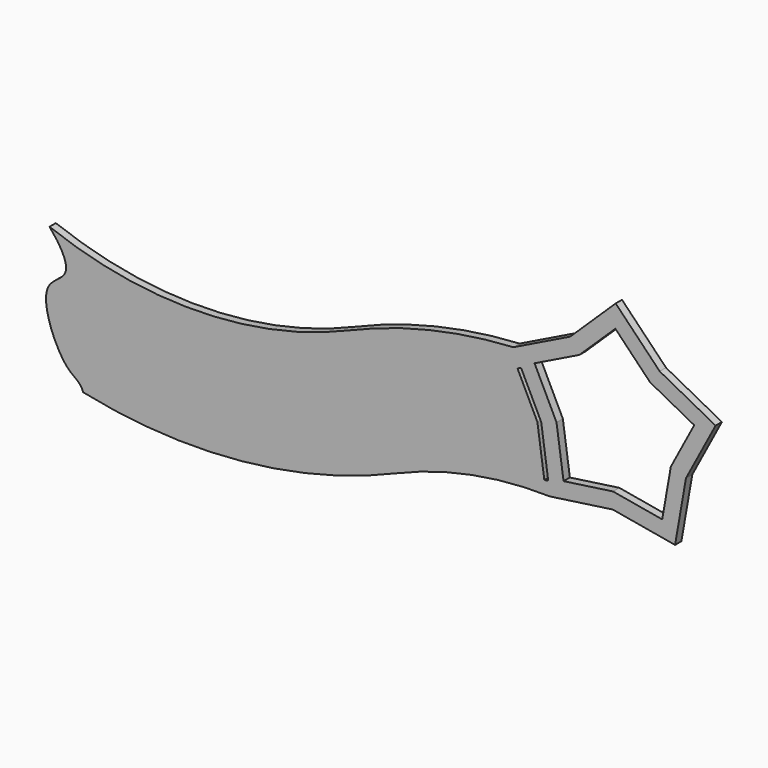
from build123d import *

# Parameters (mm, degrees)
F1_DEPTH = 3.175
F3_DEPTH = 25.4


# Not quite as in the source:
# - a feature of the source that left no trace in its solid (it failed there, or was rolled back) is left out


with BuildPart() as f1:
    # F0 (on Front) → F1 (new body)
    with BuildSketch(Plane.XZ):
        Polygon((83.7385465681, 60.7950414864), (65.4867140893, 43.1201200129), (42.6659945136, 31.9511005402), (48.4525043638, 20.1278488249), (53.8348904797, 9.1303205178), (53.9749918148, 8.1434892953), (55.6890408221, -3.9297509459), (57.4061805077, -16.0247609861), (82.5613006616, -12.4537432078), (107.5886724448, -16.8312881314), (111.9661336404, 8.1960982966), (123.863112913, 30.645911706), (101.4134680417, 42.5432090075), align=None)
        Polygon((62.8005820601, -8.8453070311), (59.98049806, 11.018507533), (51.1609480861, 29.0390003787), (69.1816050409, 37.8587515602), (83.5943604063, 51.8159429598), (97.5514190703, 37.4033246624), (115.278932926, 28.0085434102), (105.884368679, 10.2808320666), (102.427683451, -9.4821750964), (82.6646160624, -6.0254111952), align=None, mode=Mode.SUBTRACT)
        with BuildLine():
            Line((48.4525043638, 20.1278488249), (42.6659945136, 31.9511005402))
            ThreePointArc((42.6659945136, 31.9511005402), (8.9754555579, 27.0708614751), (-23.3620781244, 16.433518583))
            ThreePointArc((-23.3620781244, 16.433518583), (-83.2539454778, 3.5037557836), (-143.6249151078, 13.9708741582))
            add(Edge.make_bspline(
                [(-143.6249151078, 13.9708741582), (-139.3821490751, 9.1987873198), (-135.7140854359, 2.9639524936), (-137.4607610868, -0.5827256571), (-137.6279600012, -0.8521879559)],
                knots=[0, 0, 0, 0, 0.2240060147, 0.243416319, 0.243416319, 0.243416319, 0.243416319], degree=3))
            ThreePointArc((-137.6279600012, -0.8521879559), (-77.5676001001, -8.3586658465), (-18.6118863058, 5.3459995187))
            ThreePointArc((-18.6118863058, 5.3459995187), (14.224158407, 15.8953190594), (48.4525043638, 20.1278488249))
        make_face()
        with BuildLine():
            Line((53.8348904797, 9.1303205178), (48.4525043638, 20.1278488249))
            ThreePointArc((48.4525043638, 20.1278488249), (14.224158407, 15.8953190594), (-18.6118863058, 5.3459995187))
            ThreePointArc((-18.6118863058, 5.3459995187), (-77.5676001001, -8.3586658465), (-137.6279600012, -0.8521879559))
            add(Edge.make_bspline(
                [(-137.6279600012, -0.8521879559), (-138.9540636818, -2.9893725644), (-143.6991899879, -4.9863421871), (-144.9043234797, -9.4137473987), (-145.0020824108, -11.1490770117)],
                knots=[0.243416319, 0.243416319, 0.243416319, 0.243416319, 0.3973651411, 0.4804221604, 0.4804221604, 0.4804221604, 0.4804221604], degree=3))
            ThreePointArc((-145.0020824108, -11.1490770117), (-78.9349092151, -20.4976327315), (-13.8616894677, -5.7415173951))
            ThreePointArc((-13.8616894677, -5.7415173951), (19.3499940642, 4.6534346359), (53.9749918148, 8.1434892953))
            Line((53.9749918148, 8.1434892953), (53.8348904797, 9.1303205178))
        make_face()
        with BuildLine():
            Line((55.6890408221, -3.9297509459), (53.9749918148, 8.1434892953))
            ThreePointArc((53.9749918148, 8.1434892953), (19.3499940642, 4.6534346359), (-13.8616894677, -5.7415173951))
            ThreePointArc((-13.8616894677, -5.7415173951), (-78.9349092151, -20.4976327315), (-145.0020824108, -11.1490770117))
            add(Edge.make_bspline(
                [(-145.0020824108, -11.1490770117), (-145.148620527, -13.7502913411), (-144.2433778815, -18.4324653045), (-142.4737649258, -23.1788138286), (-141.761803512, -24.8017401992)],
                knots=[0.4804221604, 0.4804221604, 0.4804221604, 0.4804221604, 0.6049224901, 0.6738209053, 0.6738209053, 0.6738209053, 0.6738209053], degree=3))
            ThreePointArc((-141.761803512, -24.8017401992), (-74.7426386358, -32.3624002943), (-9.11149777, -16.8290365111))
            ThreePointArc((-9.11149777, -16.8290365111), (22.6146775302, -6.9930314551), (55.6890408221, -3.9297509459))
        make_face()
        with BuildLine():
            Line((57.4061805077, -16.0247609861), (55.6890408221, -3.9297509459))
            ThreePointArc((55.6890408221, -3.9297509459), (22.6146775302, -6.9930314551), (-9.11149777, -16.8290365111))
            ThreePointArc((-9.11149777, -16.8290365111), (-74.7426386358, -32.3624002943), (-141.761803512, -24.8017401992))
            add(Edge.make_bspline(
                [(-141.761803512, -24.8017401992), (-140.0858053256, -28.6222023777), (-135.8065528754, -35.5480454062), (-131.1858892441, -36.9351543486), (-130.136887087, -40.1733894927)],
                knots=[0.6738209053, 0.6738209053, 0.6738209053, 0.6738209053, 0.8360117443, 1, 1, 1, 1], degree=3))
            ThreePointArc((-130.136887087, -40.1733894927), (-66.2989601616, -43.7949576201), (-4.3613058839, -27.9165555465))
            ThreePointArc((-4.3613058839, -27.9165555465), (25.8820678715, -18.6444983253), (57.4061805077, -16.0247609861))
        make_face()
    extrude(amount=F1_DEPTH)

    # F2 (on Front) → F3 (cut)
    with BuildSketch(Plane.XZ):
        Polygon((56.6531529851, -10.7206639914), (53.8348904797, 9.1303205178), (45.7340942467, 25.6822240721), (44.3082079533, 24.9843699385), (52.2984898455, 8.6582741514), (55.0814150388, -10.9438050714), align=None)
    extrude(amount=F3_DEPTH, mode=Mode.SUBTRACT)


solid = f1.part
